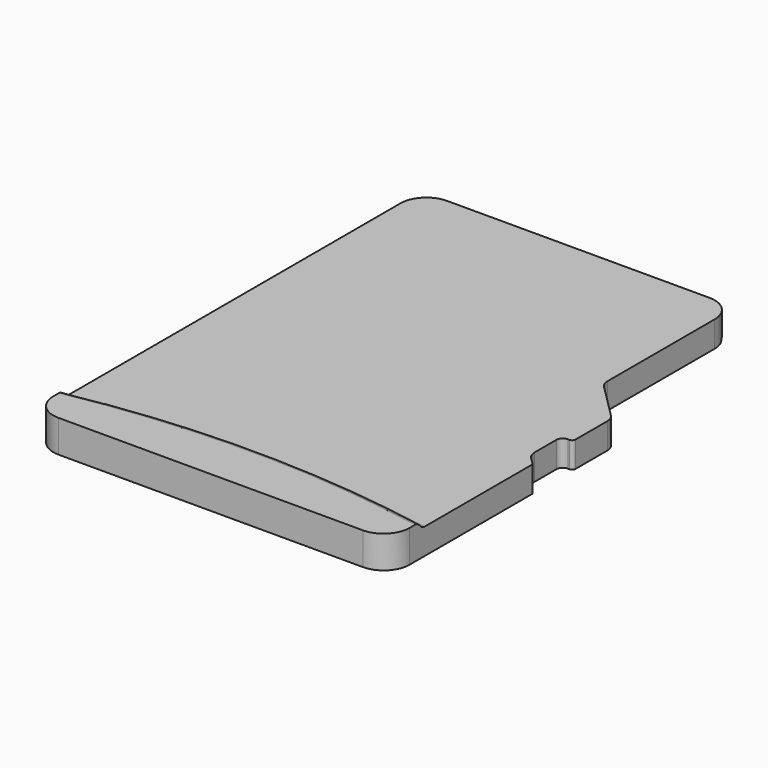
from build123d import *

# Parameters (mm, degrees)
F1_DEPTH    = 0.8
F2_DEPTH    = 1
F3_T4_ANGLE = 24.0749520294
F4_R        = 0.2
F5_T1_DEPTH = 10.790585283


# Not quite as in the source:
# - a fillet or chamfer that OpenCascade refuses, or shapes differently, is made with other operations: its cross-section is extruded or revolved along the edge and cut away or added


with BuildPart() as f1:
    # F0 (on Top) → F1 (new body)
    with BuildSketch(Plane.XY):
        with BuildLine():
            Line((-10.2, 0), (-0.8, 0))
            ThreePointArc((-0.8, 0), (-0.2343145751, 0.2343145751), (0, 0.8))
            Line((0, 0.8), (0, 0.9915242061))
            ThreePointArc((0, 0.9915242061), (-5.5, 1.5), (-11, 0.9915242061))
            Line((-11, 0.9915242061), (-11, 0.8))
            ThreePointArc((-11, 0.8), (-10.7656854249, 0.2343145751), (-10.2, 0))
        make_face()
        with BuildLine():
            ThreePointArc((-11, 0.9915242061), (-5.5, 1.5), (0, 0.9915242061))
            Line((0, 0.9915242061), (0, 1.3315242061))
            ThreePointArc((0, 1.3315242061), (-5.5, 1.84), (-11, 1.3315242061))
            Line((-11, 1.3315242061), (-11, 0.9915242061))
        make_face()
        with BuildLine():
            ThreePointArc((-11, 1.3315242061), (-5.5, 1.84), (0, 1.3315242061))
            Line((0, 1.3315242061), (0, 5.55))
            Line((0, 5.55), (-0.2328427125, 5.7828427125))
            ThreePointArc((-0.2328427125, 5.7828427125), (-0.319551813, 5.912612052), (-0.35, 6.0656854249))
            Line((-0.35, 6.0656854249), (-0.35, 6.9))
            ThreePointArc((-0.35, 6.9), (-0.2914213562, 7.0414213562), (-0.15, 7.1))
            Line((-0.15, 7.1), (-0.1, 7.1))
            ThreePointArc((-0.1, 7.1), (-0.0292893219, 7.1292893219), (0, 7.2))
            Line((0, 7.2), (0, 8.4343145751))
            ThreePointArc((0, 8.4343145751), (-0.030448187, 8.587387948), (-0.1171572875, 8.7171572875))
            Line((-0.1171572875, 8.7171572875), (-1.1828427125, 9.7828427125))
            ThreePointArc((-1.1828427125, 9.7828427125), (-1.269551813, 9.912612052), (-1.3, 10.0656854249))
            Line((-1.3, 10.0656854249), (-1.3, 14.2))
            ThreePointArc((-1.3, 14.2), (-1.5343145751, 14.7656854249), (-2.1, 15))
            Line((-2.1, 15), (-10.2, 15))
            ThreePointArc((-10.2, 15), (-10.7656854249, 14.7656854249), (-11, 14.2))
            Line((-11, 14.2), (-11, 1.3315242061))
        make_face()
    extrude(amount=F1_DEPTH)

    # F0 (on Top) → F2 (join)
    with BuildSketch(Plane.XY):
        with BuildLine():
            Line((-10.2, 0), (-0.8, 0))
            ThreePointArc((-0.8, 0), (-0.2343145751, 0.2343145751), (0, 0.8))
            Line((0, 0.8), (0, 0.9915242061))
            ThreePointArc((0, 0.9915242061), (-5.5, 1.5), (-11, 0.9915242061))
            Line((-11, 0.9915242061), (-11, 0.8))
            ThreePointArc((-11, 0.8), (-10.7656854249, 0.2343145751), (-10.2, 0))
        make_face()
    extrude(amount=F2_DEPTH)

    # F3: chamfer of 0.3 on 1 edges, made by hand


with BuildPart() as f3_tool2:
    # F3_s3 → F3_t4 (revolve)
    with BuildSketch(Plane(origin=(-11.0738065014, -2.3613816897, 0), x_dir=(0, 0, 1), z_dir=(-0.9780114007, -0.2085514329, 0))):
        Polygon((0.8, 3.5737079623), (1.1, 3.2737079623), (0.8, 3.2737079623), align=None)
    revolve(axis=Axis((-5.5, -28.5, 0.8), (0, 0, -1)), revolution_arc=F3_T4_ANGLE)

    split(bisect_by=Plane.YZ.offset(-11), keep=Keep.TOP)

    split(bisect_by=Plane.YZ, keep=Keep.BOTTOM)

    split(bisect_by=Plane.XY.offset(1), keep=Keep.BOTTOM)


with BuildPart() as f1_1:
    add(f1.part)

    # F3_t1: union F3_tool2
    add(f3_tool2.part)

    # F4
    f4_edges = [f1_1.edges().sort_by_distance(p)[0] for p in [
        (-5.5, 1.8, 0.8),
        (-5.5, 1.6, 1),
    ]]
    fillet(f4_edges, radius=F4_R)

    # F5: chamfer of 0.52 x 0.3 on 1 edges, made by hand

    # F5_s2 → F5_t1 (cut)
    with BuildSketch(Plane.YZ.offset(-11.5452926415)):
        Polygon((15, 0.3), (14.48, 0), (15, 0), align=None)
    extrude(amount=F5_T1_DEPTH, mode=Mode.SUBTRACT)


solid = f1_1.part
